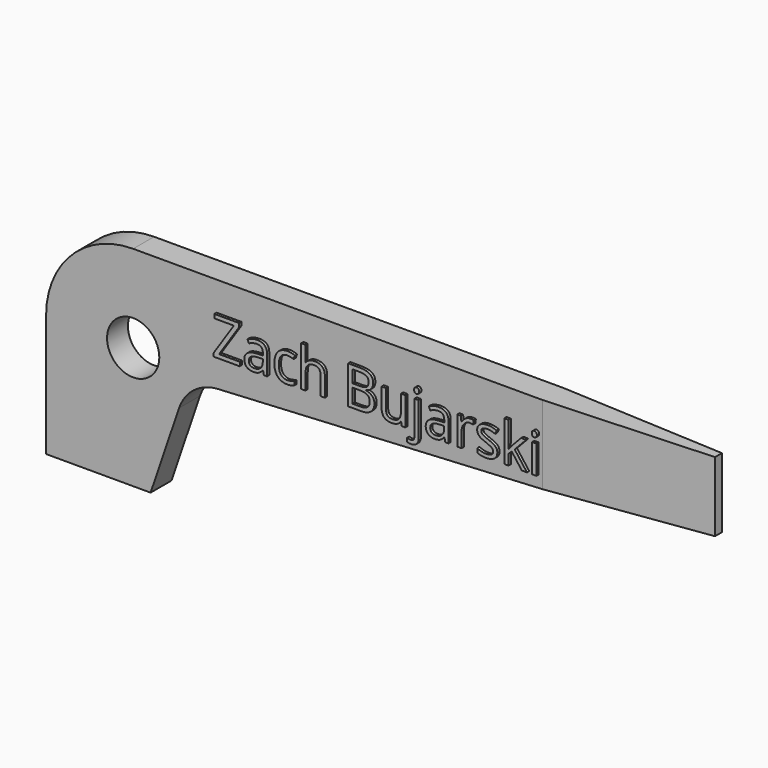
from build123d import *

# Parameters (mm, degrees)
F1_DEPTH     = 2.38125
F2_R         = 2.38125
F3_DEPTH     = 25.4
F5_DEPTH     = 25.4
F6_TEXT_SIZE = 4.8334179964
F7_DEPTH     = 0.254


# Not quite as in the source:
# - Text() gives the source's letters only with a copy of the font that has no kerning and outlines rounded to 1/6400 em; it was checked with that copy


with BuildPart() as f1:
    # F0 (on Front) → F1 (new body)
    with BuildSketch(Plane.XZ):
        with BuildLine():
            Line((60.325, 19.05), (7.9375, 19.05))
            ThreePointArc((7.9375, 19.05), (2.3248399243, 16.7251600757), (0, 11.1125))
            Line((0, 11.1125), (0, 0))
            Line((0, 0), (9.525, 0))
            Line((9.525, 0), (12.1173647876, 7.6271664624))
            ThreePointArc((12.1173647876, 7.6271664624), (13.4786145605, 9.5135918491), (15.6631963617, 10.3130942181))
            Line((15.6631963617, 10.3130942181), (60.325, 12.7))
            Line((60.325, 12.7), (60.325, 19.05))
        make_face()
    extrude(amount=F1_DEPTH)

    # F2 (on face) → F3 (cut)
    with BuildSketch(Plane.XZ.offset(2.38125)):
        with Locations((7.9375, 11.1125)):
            Circle(F2_R)
    extrude(amount=-F3_DEPTH, mode=Mode.SUBTRACT)

    # F4 (on face) → F5 (cut)
    with BuildSketch(Plane.XY.offset(19.05)):
        Polygon((60.325, -2.38125), (60.325, -1.5875), (45.24375, -2.38125), align=None)
        Polygon((60.325, 0), (45.24375, 0), (60.325, -0.79375), align=None)
    extrude(amount=-F5_DEPTH, mode=Mode.SUBTRACT)

    # F6 (on face) → F7 (join)
    with BuildSketch(Plane.XZ.offset(2.38125)):
        with Locations((15.2901524107, 12.9495738074)):
            Text('Zach Bujarski', F6_TEXT_SIZE, font='Open Sans', text_align=(TextAlign.LEFT, TextAlign.BOTTOM))
    extrude(amount=F7_DEPTH)


solid = f1.part
